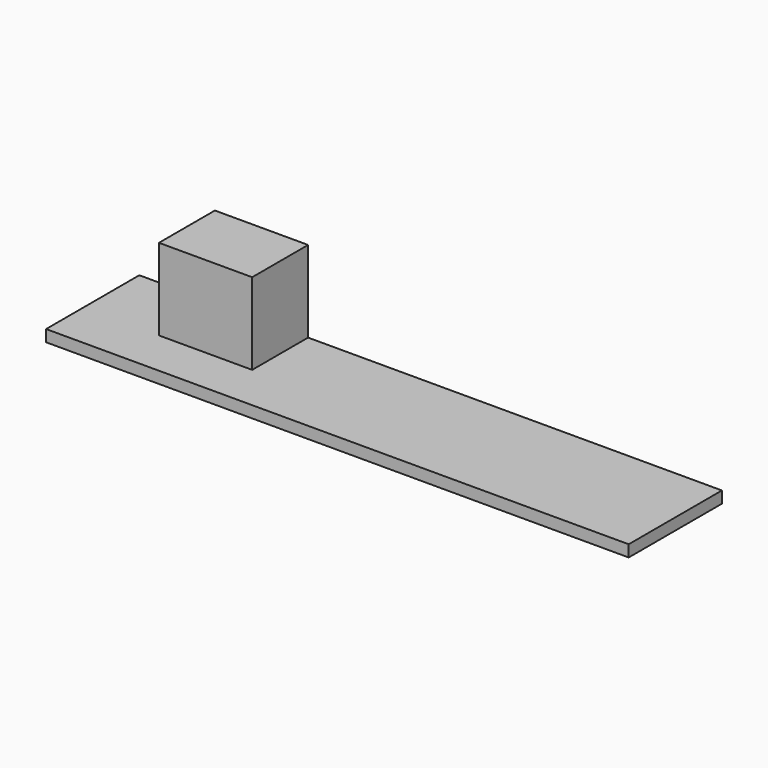
from build123d import *

# Parameters (mm, degrees)
F0_W           = 500
F0_H           = 10
F1_DEPTH       = 100
F3_E2_BOTTOM_W = 80
F3_E2_BOTTOM_H = 60
F4_DEPTH       = 80


with BuildPart() as f1:
    # F0 (on Front) → F1 (new body)
    with BuildSketch(Plane.XZ):
        with Locations((250, 5)):
            Rectangle(F0_W, F0_H)
    extrude(amount=F1_DEPTH)

    # F3_E2_bottom (on explicit) → F4 (join)
    with BuildSketch(Plane(origin=(144.8696413147, 0, 80), x_dir=(-1, 0, 0), z_dir=(0, 0, 1))):
        with Locations((40, 30)):
            Rectangle(F3_E2_BOTTOM_W, F3_E2_BOTTOM_H)
    extrude(amount=-F4_DEPTH)


solid = f1.part
